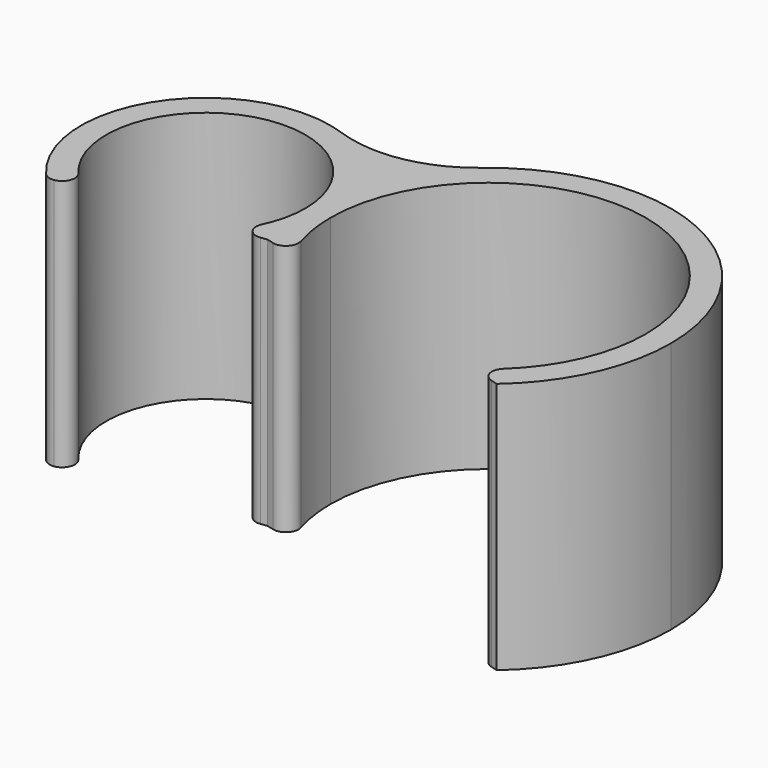
from build123d import *

# Parameters (mm, degrees)
F1_DEPTH = 10
F2_R     = 5
F3_R     = 0.49999


# Not quite as in the source:
# - a fillet or chamfer is up to 0.001 mm smaller than in the source, because OpenCascade refuses the exact size


with BuildPart() as f1:
    # F0 (on Top) → F1 (new body)
    with BuildSketch(Plane.XY):
        with BuildLine():
            ThreePointArc((-2.2598988064, -3.2396538989), (-1.8270057081, 3.5020779749), (3.95, 0))
            ThreePointArc((3.95, 0), (4.0500202922, 1.2001209016), (4.3473214286, 2.3671283017))
            ThreePointArc((4.3473214286, 2.3671283017), (-2.9159046624, 4), (-3.5838223047, -3.4144864458))
            Line((-3.5838223047, -3.4144864458), (-2.2598988064, -3.2396538989))
        make_face()
        with BuildLine():
            ThreePointArc((4.3473214286, 2.3671283017), (4.0500202922, 1.2001209016), (3.95, 0))
            ThreePointArc((3.95, 0), (4.0500202922, -1.2001209016), (4.3473214286, -2.3671283017))
            ThreePointArc((4.3473214286, -2.3671283017), (4.7969647211, -1.2213228338), (4.95, 0))
            ThreePointArc((4.95, 0), (4.7969647211, 1.2213228338), (4.3473214286, 2.3671283017))
        make_face()
        with BuildLine():
            ThreePointArc((4.3473214286, -2.3671283017), (4.0500202922, -1.2001209016), (3.95, 0))
            ThreePointArc((3.95, 0), (3.7111266365, -1.352789373), (3.0233979302, -2.5419608485))
            Line((3.0233979302, -2.5419608485), (4.3473214286, -2.3671283017))
        make_face()
        with BuildLine():
            ThreePointArc((4.95, 0), (4.7969647211, -1.2213228338), (4.3473214286, -2.3671283017))
            Line((4.3473214286, -2.3671283017), (5.5605645672, -2.6943028782))
            ThreePointArc((5.5605645672, -2.6943028782), (5.1045520487, -1.3813088983), (4.95, 0))
        make_face()
        with BuildLine():
            ThreePointArc((18.45, 0), (12.4001209016, 7.1499797078), (4.3473214286, 2.3671283017))
            ThreePointArc((4.3473214286, 2.3671283017), (4.7969647211, 1.2213228338), (4.95, 0))
            ThreePointArc((4.95, 0), (11.2, 6.25), (17.45, 0))
            ThreePointArc((17.45, 0), (16.7255629222, -2.9207284011), (14.7201905943, -5.1643739388))
            Line((14.7201905943, -5.1643739388), (15.9334337329, -5.4915485153))
            ThreePointArc((15.9334337329, -5.4915485153), (17.790898822, -3.0203563893), (18.45, 0))
        make_face()
    extrude(amount=F1_DEPTH)

    # F2
    f2_edges = [f1.edges().sort_by_distance(p)[0] for p in [
        (4.347321, 2.367128, 5),
    ]]
    fillet(f2_edges, radius=F2_R)

    # F3 (radius 0.5 in the source; OpenCascade refuses exactly that, so slightly less here)
    f3_edges = [f1.edges().sort_by_distance(p)[0] for p in [
        (-2.259899, -3.239654, 5),
        (3.023398, -2.541961, 5),
        (5.560565, -2.694303, 5),
        (14.720191, -5.164374, 5),
        (-3.583822, -3.414486, 5),
    ]]
    fillet(f3_edges, radius=F3_R)


solid = f1.part
